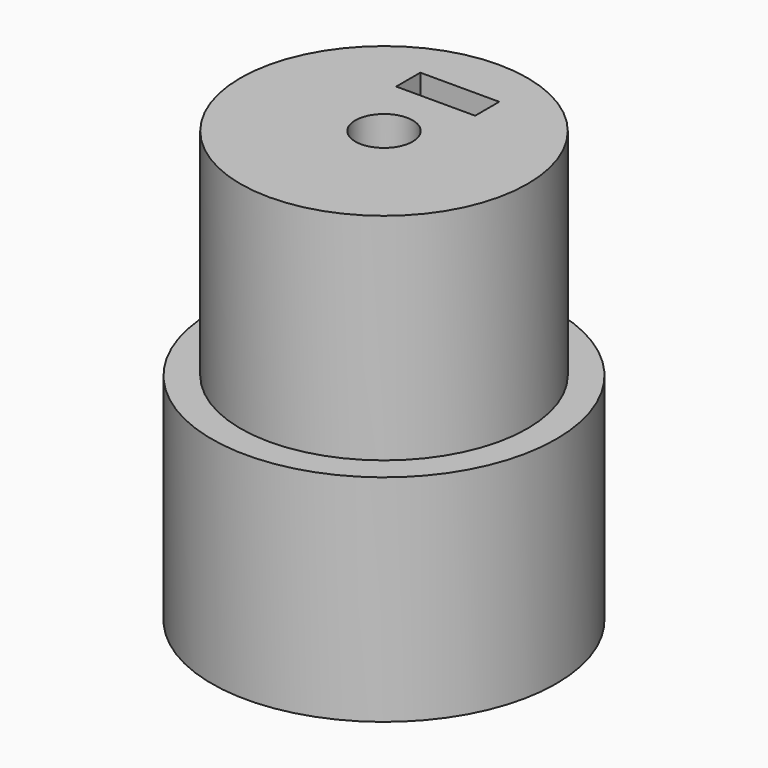
from build123d import *

# Parameters (mm, degrees)
F0_R      = 12
F0_R_2    = 6.65
F1_DEPTH  = 15
F3_R      = 1.4
F4_DEPTH  = 10
F5_R      = 10
F5_R_2    = 2
F6_DEPTH  = 15
F8_R      = 1.4
F9_DEPTH  = 11
F10_W     = 5.5
F10_H     = 2.1
F11_DEPTH = 8.5
F12_W     = 5.5
F12_H     = 2.1
F13_DEPTH = 8.5


# Not quite as in the source:
# - a feature names something its author has since deleted; it is built from what else it names


with BuildPart() as f1:
    # F0 (on Top) → F1 (new body)
    with BuildSketch(Plane.XY):
        Circle(F0_R)
        Circle(F0_R_2, mode=Mode.SUBTRACT)
    extrude(amount=F1_DEPTH)

    # F3 (on offset) → F4 (cut)
    with BuildSketch(Plane.XZ.offset(-14)):
        with Locations((0, 4)):
            Circle(F3_R)
    extrude(amount=F4_DEPTH, mode=Mode.SUBTRACT)

    # F5 (on face) → F6 (join)
    with BuildSketch(Plane.XY.offset(15)):
        Circle(F5_R)
        Circle(F5_R_2, mode=Mode.SUBTRACT)
    extrude(amount=F6_DEPTH)

    # F8 (on offset) → F9 (cut)
    with BuildSketch(Plane.XZ.offset(-11.5)):
        with Locations((0, 26)):
            Circle(F8_R)
    extrude(amount=F9_DEPTH, mode=Mode.SUBTRACT)

    # F10 (on face) → F11 (cut)
    with BuildSketch(Plane.XY.offset(30)):
        with Locations((0, 5.55)):
            Rectangle(F10_W, F10_H)
    extrude(amount=-F11_DEPTH, mode=Mode.SUBTRACT)

    # F12 (on face) → F13 (cut)
    with BuildSketch(Plane.XY):
        with Locations((0, 9.05)):
            Rectangle(F12_W, F12_H)
    extrude(amount=F13_DEPTH, mode=Mode.SUBTRACT)


solid = f1.part
